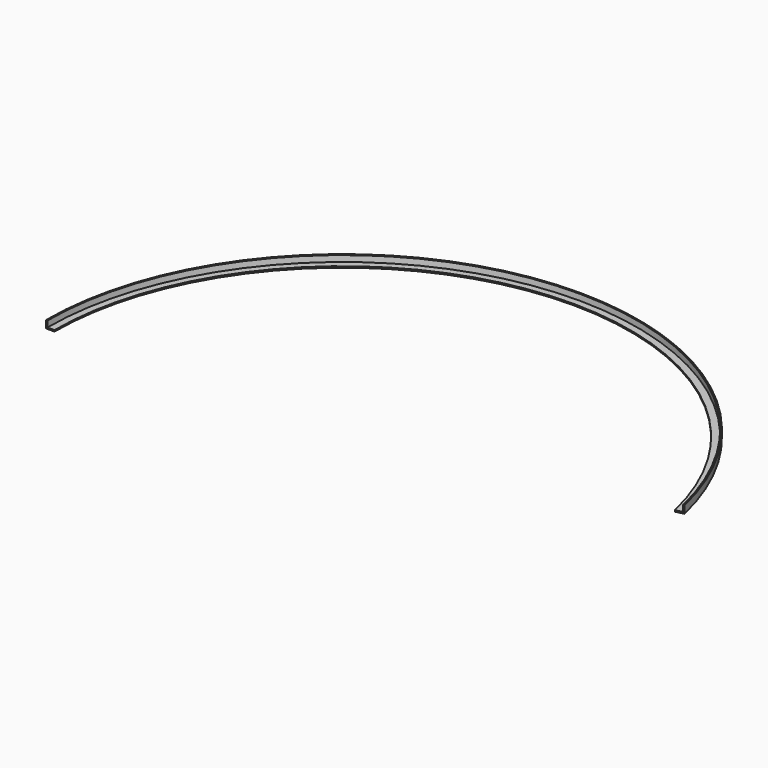
from build123d import *

# Parameters (mm, degrees)
F3_ANGLE = 167
F4_SIZE  = 1


# Not quite as in the source:
# - a feature names something its author has since deleted; it is built from what else it names


with BuildPart() as f3:
    # F2 (on Front) → F3 (revolve)
    with BuildSketch(Plane.XZ):
        Polygon((-753.25, 20), (-756.75, 20), (-756.75, 0), (-735.25, 0), (-735.25, 3.5), (-753.25, 3.5), align=None)
    revolve(axis=Axis((0, 0, 7.6849460602), (0, 0, -1)), revolution_arc=F3_ANGLE)

    # F4
    f4_edges = [f3.edges().sort_by_distance(p)[0] for p in [
        (-85.666532, 751.885502, 20),
        (-85.270321, 748.408, 20),
    ]]
    chamfer(f4_edges, length=F4_SIZE)


solid = f3.part
